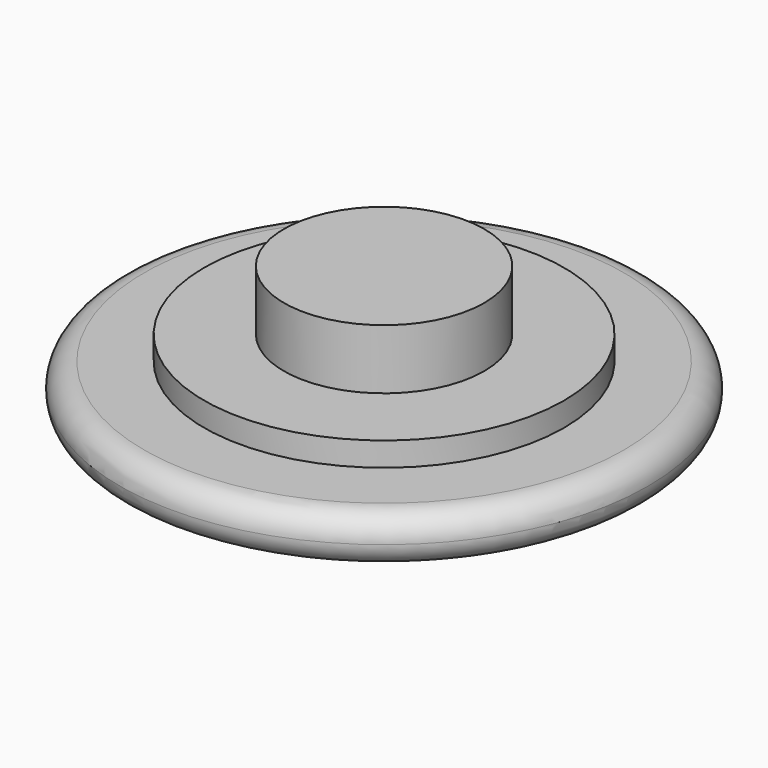
from build123d import *

# Parameters (mm, degrees)
F0_R         = 11
F0_R_2       = 7.5
F1_DEPTH     = 2
F0_R_3       = 4.175
F2_DEPTH     = 3
F3_DEPTH     = 5.5
F4_R         = 0.99999
F5_TEXT_SIZE = 5.4608181521
F6_DEPTH     = 1


# Not quite as in the source:
# - a fillet or chamfer is up to 0.001 mm smaller than in the source, because OpenCascade refuses the exact size
# - Text() gives the source's letters only with a copy of the font that has no kerning and outlines rounded to 1/6400 em; it was checked with that copy


with BuildPart() as f1:
    # F0 (on Top) → F1 (new body)
    with BuildSketch(Plane.XY):
        Circle(F0_R)
        Circle(F0_R_2, mode=Mode.SUBTRACT)
    extrude(amount=F1_DEPTH)

    # F0 (on Top) → F2 (join)
    with BuildSketch(Plane.XY):
        Circle(F0_R_2)
        Circle(F0_R_3, mode=Mode.SUBTRACT)
    extrude(amount=F2_DEPTH)

    # F0 (on Top) → F3 (join)
    with BuildSketch(Plane.XY):
        Circle(F0_R_3)
    extrude(amount=F3_DEPTH)

    # F4 (radius 1 in the source; OpenCascade refuses exactly that, so slightly less here)
    f4_edges = [f1.edges().sort_by_distance(p)[0] for p in [
        (-11, 0, 2),
        (-11, 0, 0),
    ]]
    fillet(f4_edges, radius=F4_R)

    # F5 (on face) → F6 (cut)
    with BuildSketch(Plane(origin=(0, 0, 0), x_dir=(1, 0, 0), z_dir=(0, 0, -1))):
        with Locations((-9.7947798794, -2.0155116258)):
            Text('Charley', F5_TEXT_SIZE, font='Open Sans', text_align=(TextAlign.LEFT, TextAlign.BOTTOM))
    extrude(amount=-F6_DEPTH, mode=Mode.SUBTRACT)


solid = f1.part
